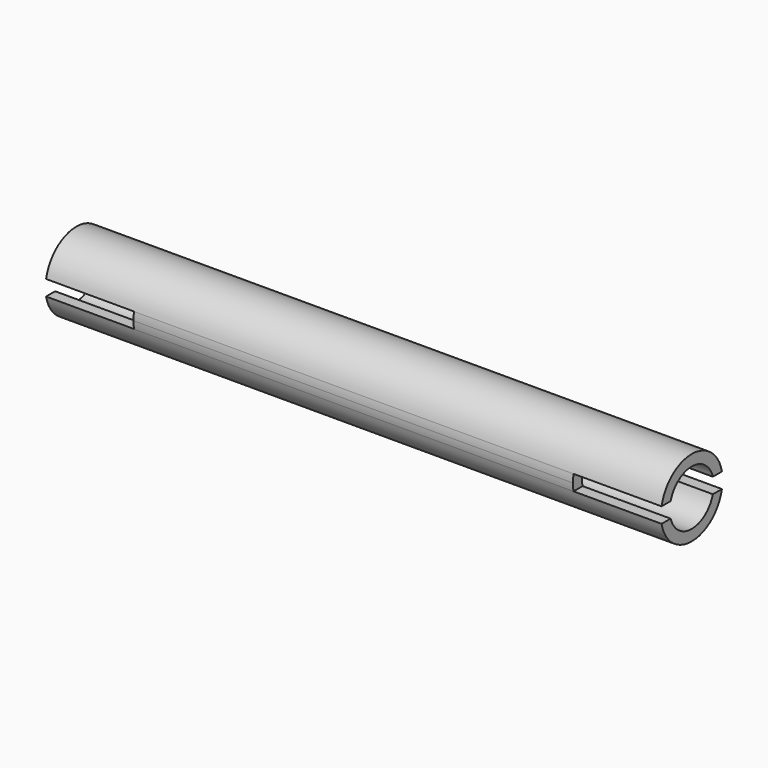
from build123d import *
from build123d import SkipClean  # not in build123d's __all__

# Parameters (mm, degrees)
F0_R          = 11.1125
F0_R_2        = 7.9375
F1_DEPTH      = 88.8365
F1_DEPTH_BACK = 88.8365
F3_DEPTH      = 177.674
F4_DEPTH      = 152.273
F5_DEPTH      = 25.4


with BuildPart() as f1:
    # F0 (on Right) → F1 (new body, two sides)
    with BuildSketch(Plane.YZ) as f1_sk:
        Circle(F0_R)
        Circle(F0_R_2, mode=Mode.SUBTRACT)
    extrude(amount=F1_DEPTH)
    extrude(f1_sk.sketch, amount=-F1_DEPTH_BACK)

    # F2 (on face) → F3 (cut, through all)
    with BuildSketch(Plane.YZ.offset(88.8365)):
        with BuildLine():
            Line((-7.62, 2.2225), (-10.8879819067, 2.2225))
            ThreePointArc((-10.8879819067, 2.2225), (-11.0562280003, 1.1169058403), (-11.1125, 0))
            ThreePointArc((-11.1125, 0), (-11.0562280003, -1.1169058403), (-10.8879819067, -2.2225))
            Line((-10.8879819067, -2.2225), (-7.62, -2.2225))
            ThreePointArc((-7.62, -2.2225), (-7.9375, 0), (-7.62, 2.2225))
        make_face()
        with BuildLine():
            ThreePointArc((11.1125, 0), (11.0562280003, 1.1169058403), (10.8879819067, 2.2225))
            Line((10.8879819067, 2.2225), (7.62, 2.2225))
            ThreePointArc((7.62, 2.2225), (7.8577241059, 1.1225320151), (7.9375, 0))
            ThreePointArc((7.9375, 0), (7.8577241059, -1.1225320151), (7.62, -2.2225))
            Line((7.62, -2.2225), (10.8879819067, -2.2225))
            ThreePointArc((10.8879819067, -2.2225), (11.0562280003, -1.1169058403), (11.1125, 0))
        make_face()
    extrude(amount=-F3_DEPTH, mode=Mode.SUBTRACT)

    # F2 (on face) → F4 (join)
    with BuildSketch(Plane.YZ.offset(88.8365)):
        with BuildLine():
            Line((-7.62, 2.2225), (-10.8879819067, 2.2225))
            ThreePointArc((-10.8879819067, 2.2225), (-11.0562280003, 1.1169058403), (-11.1125, 0))
            ThreePointArc((-11.1125, 0), (-11.0562280003, -1.1169058403), (-10.8879819067, -2.2225))
            Line((-10.8879819067, -2.2225), (-7.62, -2.2225))
            ThreePointArc((-7.62, -2.2225), (-7.9375, 0), (-7.62, 2.2225))
        make_face()
        with BuildLine():
            ThreePointArc((11.1125, 0), (11.0562280003, 1.1169058403), (10.8879819067, 2.2225))
            Line((10.8879819067, 2.2225), (7.62, 2.2225))
            ThreePointArc((7.62, 2.2225), (7.8577241059, 1.1225320151), (7.9375, 0))
            ThreePointArc((7.9375, 0), (7.8577241059, -1.1225320151), (7.62, -2.2225))
            Line((7.62, -2.2225), (10.8879819067, -2.2225))
            ThreePointArc((10.8879819067, -2.2225), (11.0562280003, -1.1169058403), (11.1125, 0))
        make_face()
    with SkipClean():  # cleaning this boolean's faces spoils the solid; the shape is the same uncleaned
        extrude(amount=-F4_DEPTH)

    # F2 (on face) → F5 (cut)
    with BuildSketch(Plane.YZ.offset(88.8365)):
        with BuildLine():
            Line((-7.62, 2.2225), (-10.8879819067, 2.2225))
            ThreePointArc((-10.8879819067, 2.2225), (-11.0562280003, 1.1169058403), (-11.1125, 0))
            ThreePointArc((-11.1125, 0), (-11.0562280003, -1.1169058403), (-10.8879819067, -2.2225))
            Line((-10.8879819067, -2.2225), (-7.62, -2.2225))
            ThreePointArc((-7.62, -2.2225), (-7.9375, 0), (-7.62, 2.2225))
        make_face()
        with BuildLine():
            ThreePointArc((11.1125, 0), (11.0562280003, 1.1169058403), (10.8879819067, 2.2225))
            Line((10.8879819067, 2.2225), (7.62, 2.2225))
            ThreePointArc((7.62, 2.2225), (7.8577241059, 1.1225320151), (7.9375, 0))
            ThreePointArc((7.9375, 0), (7.8577241059, -1.1225320151), (7.62, -2.2225))
            Line((7.62, -2.2225), (10.8879819067, -2.2225))
            ThreePointArc((10.8879819067, -2.2225), (11.0562280003, -1.1169058403), (11.1125, 0))
        make_face()
    with SkipClean():  # cleaning this boolean's faces spoils the solid; the shape is the same uncleaned
        extrude(amount=-F5_DEPTH, mode=Mode.SUBTRACT)


solid = f1.part
